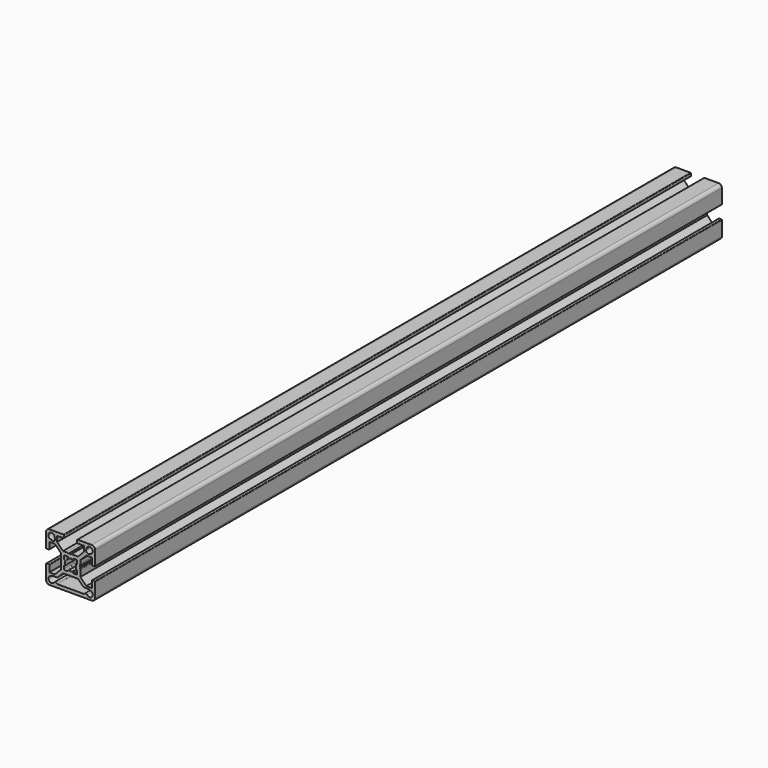
from build123d import *

# Parameters (mm, degrees)
F2_DEPTH = 240


# Not quite as in the source:
# - ends of sketch curves that miss each other by under 0.0002 mm in the source are joined


with BuildPart() as f2:
    # F1 (on Front) → F2 (new body, symmetric)
    with BuildSketch(Plane.XZ):
        with BuildLine():
            Line((8.249944, 9.6642), (4.58573, 5.999986))
            Line((4.58573, 5.999986), (0.653534, 5.999986))
            ThreePointArc((0.653534, 5.999986), (0.5241245494, 5.9829489324), (0.4035341291, 5.9329987764))
            Line((0.4035341291, 5.9329987764), (-5.6e-05, 5.699986))
            Line((-5.6e-05, 5.699986), (-0.403646, 5.932999))
            ThreePointArc((-0.403646, 5.932999), (-0.653646, 5.999986), (-0.9036458709, 5.9329987764))
            Line((-0.9036458709, 5.9329987764), (-1.218942, 5.750963))
            Line((-1.218942, 5.750963), (-2.500056, 5.999986))
            Line((-2.500056, 5.999986), (-4.585842, 5.999986))
            Line((-4.585842, 5.999986), (-8.250056, 9.6642))
            Line((-8.250056, 9.6642), (-8.250056, 12.999986))
            Line((-8.250056, 12.999986), (-4.300056, 12.999986))
            ThreePointArc((-4.300056, 12.999986), (-4.0879239656, 13.0878539656), (-4.000056, 13.299986))
            Line((-4.000056, 13.299986), (-4.000056, 14.699986))
            ThreePointArc((-4.000056, 14.699986), (-4.0879239656, 14.9121180344), (-4.300056, 14.999986))
            Line((-4.300056, 14.999986), (-13.000056, 14.999986))
            ThreePointArc((-13.000056, 14.999986), (-14.4142695624, 14.4141995624), (-15.000056, 12.999986))
            Line((-15.000056, 12.999986), (-15.000056, 4.299986))
            ThreePointArc((-15.000056, 4.299986), (-14.9121880344, 4.0878539656), (-14.700056, 3.999986))
            Line((-14.700056, 3.999986), (-13.300056, 3.999986))
            ThreePointArc((-13.300056, 3.999986), (-13.0879239656, 4.0878539656), (-13.000056, 4.299986))
            Line((-13.000056, 4.299986), (-13.000056, 8.249986))
            Line((-13.000056, 8.249986), (-9.66427, 8.249986))
            Line((-9.66427, 8.249986), (-6.000056, 4.585772))
            Line((-6.000056, 4.585772), (-6.000056, 0.653576))
            ThreePointArc((-6.000056, 0.653576), (-5.9830189324, 0.5241665494), (-5.9330687764, 0.4035761291))
            Line((-5.9330687764, 0.4035761291), (-5.700056, -1.4e-05))
            Line((-5.700056, -1.4e-05), (-5.933069, -0.403604))
            ThreePointArc((-5.933069, -0.403604), (-6.000056, -0.653604), (-5.9330687764, -0.9036038709))
            Line((-5.9330687764, -0.9036038709), (-5.751033, -1.2189))
            Line((-5.751033, -1.2189), (-6.000056, -2.500014))
            Line((-6.000056, -2.500014), (-6.000056, -4.5858))
            Line((-6.000056, -4.5858), (-9.66427, -8.250014))
            Line((-9.66427, -8.250014), (-13.000056, -8.250014))
            Line((-13.000056, -8.250014), (-13.000056, -4.300014))
            ThreePointArc((-13.000056, -4.300014), (-13.0879239656, -4.0878819656), (-13.300056, -4.000014))
            Line((-13.300056, -4.000014), (-14.700056, -4.000014))
            ThreePointArc((-14.700056, -4.000014), (-14.9121880344, -4.0878819656), (-15.000056, -4.300014))
            Line((-15.000056, -4.300014), (-15.000056, -13.000014))
            ThreePointArc((-15.000056, -13.000014), (-14.4142695624, -14.4142275624), (-13.000056, -15.000014))
            Line((-13.000056, -15.000014), (12.999944, -15.000014))
            ThreePointArc((12.999944, -15.000014), (14.4141575624, -14.4142275624), (14.999944, -13.000014))
            Line((14.999944, -13.000014), (14.999944, -4.300014))
            ThreePointArc((14.999944, -4.300014), (14.9120760344, -4.0878819656), (14.699944, -4.000014))
            Line((14.699944, -4.000014), (13.299944, -4.000014))
            ThreePointArc((13.299944, -4.000014), (13.0878119656, -4.0878819656), (12.999944, -4.300014))
            Line((12.999944, -4.300014), (12.999944, -8.250014))
            Line((12.999944, -8.250014), (9.664158, -8.250014))
            Line((9.664158, -8.250014), (5.999944, -4.5858))
            Line((5.999944, -4.5858), (5.999944, -0.653604))
            ThreePointArc((5.999944, -0.653604), (5.9829069324, -0.5241945494), (5.9329567764, -0.4036041291))
            Line((5.9329567764, -0.4036041291), (5.699944, -1.4e-05))
            Line((5.699944, -1.4e-05), (5.932957, 0.403576))
            ThreePointArc((5.932957, 0.403576), (5.999944, 0.653576), (5.9329567764, 0.9035758709))
            Line((5.9329567764, 0.9035758709), (5.750921, 1.218872))
            Line((5.750921, 1.218872), (5.999944, 2.499986))
            Line((5.999944, 2.499986), (5.999944, 4.585772))
            Line((5.999944, 4.585772), (9.664158, 8.249986))
            Line((9.664158, 8.249986), (12.999944, 8.249986))
            Line((12.999944, 8.249986), (12.999944, 4.299986))
            ThreePointArc((12.999944, 4.299986), (13.0878119656, 4.0878539656), (13.299944, 3.999986))
            Line((13.299944, 3.999986), (14.699944, 3.999986))
            ThreePointArc((14.699944, 3.999986), (14.9120760344, 4.0878539656), (14.999944, 4.299986))
            Line((14.999944, 4.299986), (14.999944, 12.999986))
            ThreePointArc((14.999944, 12.999986), (14.4141575624, 14.4141995624), (12.999944, 14.999986))
            Line((12.999944, 14.999986), (4.299944, 14.999986))
            ThreePointArc((4.299944, 14.999986), (4.0878119656, 14.9121180344), (3.999944, 14.699986))
            Line((3.999944, 14.699986), (3.999944, 13.299986))
            ThreePointArc((3.999944, 13.299986), (4.0878119656, 13.0878539656), (4.299944, 12.999986))
            Line((4.299944, 12.999986), (8.249944, 12.999986))
            Line((8.249944, 12.999986), (8.249944, 9.6642))
        make_face()
        with BuildLine():
            Line((-4.171629, -6.000014), (4.171517, -6.000014))
            ThreePointArc((4.171517, -6.000014), (4.5542004324, -6.0761344675), (4.8786237812, -6.2929072188))
            Line((4.8786237812, -6.2929072188), (7.742837, -9.157121))
            ThreePointArc((7.742837, -9.157121), (8.0672605676, -9.3738935325), (8.449944, -9.450014))
            Line((8.449944, -9.450014), (11.073348, -9.450014))
            Line((11.073348, -9.450014), (12.349782, -9.914598))
            ThreePointArc((12.349782, -9.914598), (13.2040603505, -12.8608903949), (10.1374570291, -12.7810479799))
            ThreePointArc((10.1374570291, -12.7810479799), (9.3136995047, -12.3500149751), (8.4911490608, -12.7833470418))
            ThreePointArc((8.4911490608, -12.7833470418), (8.3119125635, -12.9425444809), (8.079175, -13.000014))
            Line((8.079175, -13.000014), (-8.079287, -13.000014))
            ThreePointArc((-8.079287, -13.000014), (-8.3120245635, -12.9425444809), (-8.4912608636, -12.7833469062))
            ThreePointArc((-8.4912608636, -12.7833469062), (-9.3138115047, -12.3500149751), (-10.1375690315, -12.7810479782))
            ThreePointArc((-10.1375690315, -12.7810479782), (-13.2041723505, -12.8608903949), (-12.3498940253, -9.9145979306))
            Line((-12.3498940253, -9.9145979306), (-11.07346, -9.450014))
            Line((-11.07346, -9.450014), (-8.450056, -9.450014))
            ThreePointArc((-8.450056, -9.450014), (-8.0673725676, -9.3738935325), (-7.7429492188, -9.1571207812))
            Line((-7.7429492188, -9.1571207812), (-4.878736, -6.292907))
            ThreePointArc((-4.878736, -6.292907), (-4.5543124324, -6.0761344675), (-4.171629, -6.000014))
        make_face(mode=Mode.SUBTRACT)
        with BuildLine():
            ThreePointArc((-12.3498940253, 9.9145699306), (-13.0435588843, 13.0434888843), (-9.9146399306, 12.3498240253))
            Line((-9.9146399306, 12.3498240253), (-9.547908, 11.342236))
            ThreePointArc((-9.547908, 11.342236), (-9.8735275063, 9.8734575063), (-11.3423061215, 9.5478376661))
            Line((-11.3423061215, 9.5478376661), (-12.3498940253, 9.9145699306))
        make_face(mode=Mode.SUBTRACT)
        with BuildLine():
            ThreePointArc((0.9882629956, -3.2532009855), (-5.6e-05, -3.400014), (-0.9883749956, -3.2532009855))
            ThreePointArc((-0.9883749956, -3.2532009855), (-1.3178396431, -3.2974811593), (-1.5000564258, -3.5755229349))
            ThreePointArc((-1.5000564258, -3.5755229349), (-1.6685571025, -3.8793255231), (-1.994322, -4.000014))
            Line((-1.994322, -4.000014), (-3.500056, -4.000014))
            ThreePointArc((-3.500056, -4.000014), (-3.8536093906, -3.8535673906), (-4.000056, -3.500014))
            Line((-4.000056, -3.500014), (-4.000056, -1.99428))
            ThreePointArc((-4.000056, -1.99428), (-3.8793675231, -1.6685151025), (-3.5755649263, -1.5000144822))
            ThreePointArc((-3.5755649263, -1.5000144822), (-3.2975231593, -1.3177976431), (-3.2532441585, -0.9883290481))
            ThreePointArc((-3.2532441585, -0.9883290481), (-3.400056, -1.4e-05), (-3.2532429855, 0.9883049956))
            ThreePointArc((-3.2532429855, 0.9883049956), (-3.2975231593, 1.3177696431), (-3.5755649349, 1.4999864258))
            ThreePointArc((-3.5755649349, 1.4999864258), (-3.8793675231, 1.6684871025), (-4.000056, 1.994252))
            Line((-4.000056, 1.994252), (-4.000056, 3.499986))
            ThreePointArc((-4.000056, 3.499986), (-3.8536093906, 3.8535393906), (-3.500056, 3.999986))
            Line((-3.500056, 3.999986), (-1.994322, 3.999986))
            ThreePointArc((-1.994322, 3.999986), (-1.6685571025, 3.8792975231), (-1.5000564822, 3.5754949263))
            ThreePointArc((-1.5000564822, 3.5754949263), (-1.3178396431, 3.2974531593), (-0.9883710481, 3.2531741585))
            ThreePointArc((-0.9883710481, 3.2531741585), (-5.6e-05, 3.399986), (0.9882629956, 3.2531729855))
            ThreePointArc((0.9882629956, 3.2531729855), (1.3177276431, 3.2974531593), (1.4999444258, 3.5754949349))
            ThreePointArc((1.4999444258, 3.5754949349), (1.6684451025, 3.8792975231), (1.99421, 3.999986))
            Line((1.99421, 3.999986), (3.499944, 3.999986))
            ThreePointArc((3.499944, 3.999986), (3.8534973906, 3.8535393906), (3.999944, 3.499986))
            Line((3.999944, 3.499986), (3.999944, 1.994252))
            ThreePointArc((3.999944, 1.994252), (3.8792555231, 1.6684871025), (3.5754529263, 1.4999864822))
            ThreePointArc((3.5754529263, 1.4999864822), (3.2974111593, 1.3177696431), (3.2531321585, 0.9883010481))
            ThreePointArc((3.2531321585, 0.9883010481), (3.399944, -1.4e-05), (3.2531309855, -0.9883329956))
            ThreePointArc((3.2531309855, -0.9883329956), (3.2974111593, -1.3177976431), (3.5754529349, -1.5000144258))
            ThreePointArc((3.5754529349, -1.5000144258), (3.8792555231, -1.6685151025), (3.999944, -1.99428))
            Line((3.999944, -1.99428), (3.999944, -3.500014))
            ThreePointArc((3.999944, -3.500014), (3.8534973906, -3.8535673906), (3.499944, -4.000014))
            Line((3.499944, -4.000014), (1.99421, -4.000014))
            ThreePointArc((1.99421, -4.000014), (1.6684451025, -3.8793255231), (1.4999444822, -3.5755229263))
            ThreePointArc((1.4999444822, -3.5755229263), (1.3177276431, -3.2974811593), (0.9882629956, -3.2532009855))
        make_face(mode=Mode.SUBTRACT)
        with BuildLine():
            ThreePointArc((11.3421941215, 9.5478376661), (9.8734155063, 9.8734575063), (9.5477956661, 11.3422361215))
            Line((9.5477956661, 11.3422361215), (9.914528, 12.349824))
            ThreePointArc((9.914528, 12.349824), (13.0434468843, 13.0434888843), (12.3497820253, 9.9145699306))
            Line((12.3497820253, 9.9145699306), (11.3421941215, 9.5478376661))
        make_face(mode=Mode.SUBTRACT)
    extrude(amount=F2_DEPTH, both=True)


solid = f2.part
